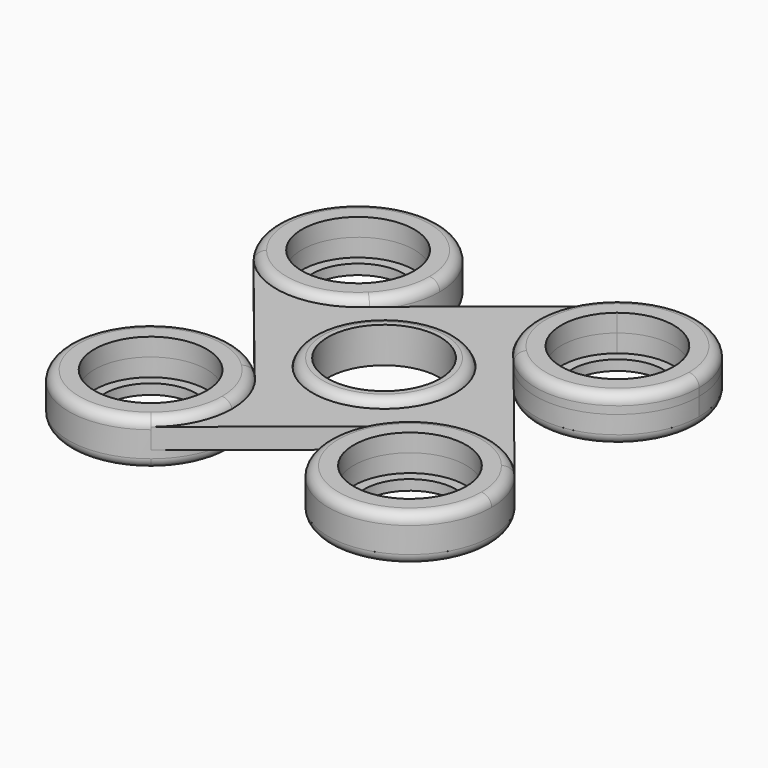
from build123d import *

# Parameters (mm, degrees)
F0_R     = 14
F1_DEPTH = 2
F2_DEPTH = 3.5
F3_R     = 9
F4_DEPTH = 2
F3_R_2   = 16
F0_R_2   = 11
F5_DEPTH = 3.5
F6_R     = 1.99999
F6_2_R   = 1.99999
F6_3_R   = 1.99999
F6_4_R   = 1.99999
F6_5_R   = 1.99999
F6_6_R   = 1.99999
F6_7_R   = 1.99999
F6_8_R   = 1.99999
F6_9_R   = 1.99999


# Not quite as in the source:
# - a fillet or chamfer is up to 0.001 mm smaller than in the source, because OpenCascade refuses the exact size


with BuildPart() as f1:
    # F0 (on Top) → F1 (new body, symmetric)
    with BuildSketch(Plane.XY):
        with BuildLine():
            ThreePointArc((11.313708499, -11.313708499), (-0.8494425911, -15.9774355666), (-12.4495307232, -10.0503325703))
            Line((-12.4495307232, -10.0503325703), (11.313708499, -39.486291501))
            ThreePointArc((11.313708499, -39.486291501), (14.7820725202, -44.6770650822), (16, -50.8))
            ThreePointArc((16, -50.8), (14.4361580956, -57.699082507), (10.0503325703, -63.2495307232))
            Line((10.0503325703, -63.2495307232), (39.486291501, -39.486291501))
            ThreePointArc((39.486291501, -39.486291501), (51.6494425911, -34.8225644334), (63.2495307232, -40.7496674297))
            Line((63.2495307232, -40.7496674297), (39.486291501, -11.313708499))
            ThreePointArc((39.486291501, -11.313708499), (34.8225644334, 0.8494425911), (40.7496674297, 12.4495307232))
            Line((40.7496674297, 12.4495307232), (11.313708499, -11.313708499))
        make_face()
        with Locations((25.4, -25.4)):
            Circle(F0_R, mode=Mode.SUBTRACT)
    extrude(amount=F1_DEPTH, both=True)


with BuildPart() as f2:
    # F0 (on Top) → F2 (new body, symmetric)
    with BuildSketch(Plane.XY):
        with BuildLine():
            ThreePointArc((16, -50.8), (14.7820725202, -44.6770650822), (11.313708499, -39.486291501))
            ThreePointArc((11.313708499, -39.486291501), (-15.9774355666, -49.9505574089), (10.0503325703, -63.2495307232))
            ThreePointArc((10.0503325703, -63.2495307232), (14.4361580956, -57.699082507), (16, -50.8))
        make_face()
        with BuildLine():
            ThreePointArc((11, -50.8), (9.9248586907, -55.5431192235), (6.909603642, -59.3590523722))
            ThreePointArc((6.909603642, -59.3590523722), (-9.9248586907, -46.0568807765), (11, -50.8))
        make_face(mode=Mode.SUBTRACT)
    extrude(amount=F2_DEPTH, both=True)

    # F6 (radius 2 in the source; OpenCascade refuses exactly that, so slightly less here)
    f6_edges = [f2.edges().sort_by_distance(p)[0] for p in [
        (-15.977436, -49.950557, 3.5),
    ]]
    fillet(f6_edges, radius=F6_R)


with BuildPart() as f2b:
    # F0 (on Top) → F2, piece 2 (new body, symmetric)
    with BuildSketch(Plane.XY):
        with BuildLine():
            ThreePointArc((63.2495307232, -40.7496674297), (51.6494425911, -34.8225644334), (39.486291501, -39.486291501))
            ThreePointArc((39.486291501, -39.486291501), (44.6770650822, -65.5820725202), (66.8, -50.8))
            ThreePointArc((66.8, -50.8), (65.8862933083, -45.4704827409), (63.2495307232, -40.7496674297))
        make_face()
        with BuildLine():
            ThreePointArc((61.8, -50.8), (40.4281733505, -54.4640431156), (59.3590523722, -43.890396358))
            ThreePointArc((59.3590523722, -43.890396358), (61.1718266495, -47.1359568844), (61.8, -50.8))
        make_face(mode=Mode.SUBTRACT)
    extrude(amount=F2_DEPTH, both=True)

    # F6#4 (radius 2 in the source; OpenCascade refuses exactly that, so slightly less here)
    f6_4_edges = [f2b.edges().sort_by_distance(p)[0] for p in [
        (44.677065, -65.582073, 3.5),
    ]]
    fillet(f6_4_edges, radius=F6_4_R)


with BuildPart() as f2c:
    # F0 (on Top) → F2, piece 3 (new body, symmetric)
    with BuildSketch(Plane.XY):
        with BuildLine():
            ThreePointArc((66.8, 0), (57.699082507, 14.4361580956), (40.7496674297, 12.4495307232))
            ThreePointArc((40.7496674297, 12.4495307232), (34.8225644334, 0.8494425911), (39.486291501, -11.313708499))
            ThreePointArc((39.486291501, -11.313708499), (56.9229349178, -14.7820725202), (66.8, 0))
        make_face()
        with BuildLine():
            ThreePointArc((61.8, 0), (46.0568807765, -9.9248586907), (43.890396358, 8.5590523722))
            ThreePointArc((43.890396358, 8.5590523722), (55.5431192235, 9.9248586907), (61.8, 0))
        make_face(mode=Mode.SUBTRACT)
    extrude(amount=F2_DEPTH, both=True)

    # F6#6 (radius 2 in the source; OpenCascade refuses exactly that, so slightly less here)
    f6_6_edges = [f2c.edges().sort_by_distance(p)[0] for p in [
        (34.822564, 0.849443, 3.5),
    ]]
    fillet(f6_6_edges, radius=F6_6_R)


with BuildPart() as f2d:
    # F0 (on Top) → F2, piece 4 (new body, symmetric)
    with BuildSketch(Plane.XY):
        with BuildLine():
            ThreePointArc((16, 0), (-5.3295172591, 15.0862933083), (-12.4495307232, -10.0503325703))
            ThreePointArc((-12.4495307232, -10.0503325703), (-0.8494425911, -15.9774355666), (11.313708499, -11.313708499))
            ThreePointArc((11.313708499, -11.313708499), (14.7820725202, -6.1229349178), (16, 0))
        make_face()
        with BuildLine():
            ThreePointArc((-8.5590523722, -6.909603642), (-3.6640431156, 10.3718266495), (11, 0))
            ThreePointArc((11, 0), (3.6640431156, -10.3718266495), (-8.5590523722, -6.909603642))
        make_face(mode=Mode.SUBTRACT)
    extrude(amount=F2_DEPTH, both=True)

    # F6#8 (radius 2 in the source; OpenCascade refuses exactly that, so slightly less here)
    f6_8_edges = [f2d.edges().sort_by_distance(p)[0] for p in [
        (-5.329517, 15.086293, 3.5),
    ]]
    fillet(f6_8_edges, radius=F6_8_R)


with BuildPart() as f4:
    # F3 (on face) → F4 (new body)
    with BuildSketch(Plane(origin=(0, 0, -3.5), x_dir=(1, 0, 0), z_dir=(0, 0, -1))):
        with BuildLine():
            ThreePointArc((11.313708499, 39.486291501), (14.7820725202, 44.6770650822), (16, 50.8))
            ThreePointArc((16, 50.8), (14.4361580956, 57.699082507), (10.0503325703, 63.2495307232))
            ThreePointArc((10.0503325703, 63.2495307232), (-15.9774355666, 49.9505574089), (11.313708499, 39.486291501))
        make_face()
        with BuildLine():
            ThreePointArc((11, 50.8), (-9.9248586907, 46.0568807765), (6.909603642, 59.3590523722))
            ThreePointArc((6.909603642, 59.3590523722), (9.9248586907, 55.5431192235), (11, 50.8))
        make_face(mode=Mode.SUBTRACT)
        with BuildLine():
            ThreePointArc((11, 50.8), (9.9248586907, 55.5431192235), (6.909603642, 59.3590523722))
            ThreePointArc((6.909603642, 59.3590523722), (-9.9248586907, 46.0568807765), (11, 50.8))
        make_face()
        with Locations((0, 50.8)):
            Circle(F3_R, mode=Mode.SUBTRACT)
    extrude(amount=F4_DEPTH)

    # F6#2 (radius 2 in the source; OpenCascade refuses exactly that, so slightly less here)
    f6_2_edges = [f4.edges().sort_by_distance(p)[0] for p in [
        (-16, -50.8, -5.5),
    ]]
    fillet(f6_2_edges, radius=F6_2_R)


with BuildPart() as f4b:
    # F3 (on face) → F4, piece 2 (new body)
    with BuildSketch(Plane(origin=(0, 0, -3.5), x_dir=(1, 0, 0), z_dir=(0, 0, -1))):
        with Locations((50.8, 50.8)):
            Circle(F3_R_2)
        with Locations((50.8, 50.8)):
            Circle(F3_R, mode=Mode.SUBTRACT)
    extrude(amount=F4_DEPTH)

    # F6#3 (radius 2 in the source; OpenCascade refuses exactly that, so slightly less here)
    f6_3_edges = [f4b.edges().sort_by_distance(p)[0] for p in [
        (34.8, -50.8, -5.5),
    ]]
    fillet(f6_3_edges, radius=F6_3_R)


with BuildPart() as f4c:
    # F3 (on face) → F4, piece 3 (new body)
    with BuildSketch(Plane(origin=(0, 0, -3.5), x_dir=(1, 0, 0), z_dir=(0, 0, -1))):
        with Locations((50.8, 0)):
            Circle(F3_R_2)
        with Locations((50.8, 0)):
            Circle(F3_R, mode=Mode.SUBTRACT)
    extrude(amount=F4_DEPTH)

    # F6#5 (radius 2 in the source; OpenCascade refuses exactly that, so slightly less here)
    f6_5_edges = [f4c.edges().sort_by_distance(p)[0] for p in [
        (34.8, 0, -5.5),
    ]]
    fillet(f6_5_edges, radius=F6_5_R)


with BuildPart() as f4d:
    # F3 (on face) → F4, piece 4 (new body)
    with BuildSketch(Plane(origin=(0, 0, -3.5), x_dir=(1, 0, 0), z_dir=(0, 0, -1))):
        Circle(F3_R_2)
        Circle(F3_R, mode=Mode.SUBTRACT)
    extrude(amount=F4_DEPTH)

    # F6#7 (radius 2 in the source; OpenCascade refuses exactly that, so slightly less here)
    f6_7_edges = [f4d.edges().sort_by_distance(p)[0] for p in [
        (-16, 0, -5.5),
    ]]
    fillet(f6_7_edges, radius=F6_7_R)


with BuildPart() as f5:
    # F0 (on Top) → F5 (new body, symmetric)
    with BuildSketch(Plane.XY):
        with Locations((25.4, -25.4)):
            Circle(F0_R)
        with Locations((25.4, -25.4)):
            Circle(F0_R_2, mode=Mode.SUBTRACT)
    extrude(amount=F5_DEPTH, both=True)

    # F6#9 (radius 2 in the source; OpenCascade refuses exactly that, so slightly less here)
    f6_9_edges = [f5.edges().sort_by_distance(p)[0] for p in [
        (11.4, -25.4, 3.5),
        (11.4, -25.4, -3.5),
    ]]
    fillet(f6_9_edges, radius=F6_9_R)


solid = Compound([f1.part, f2.part, f2b.part, f2c.part, f2d.part, f4.part, f4b.part, f4c.part, f4d.part, f5.part])
